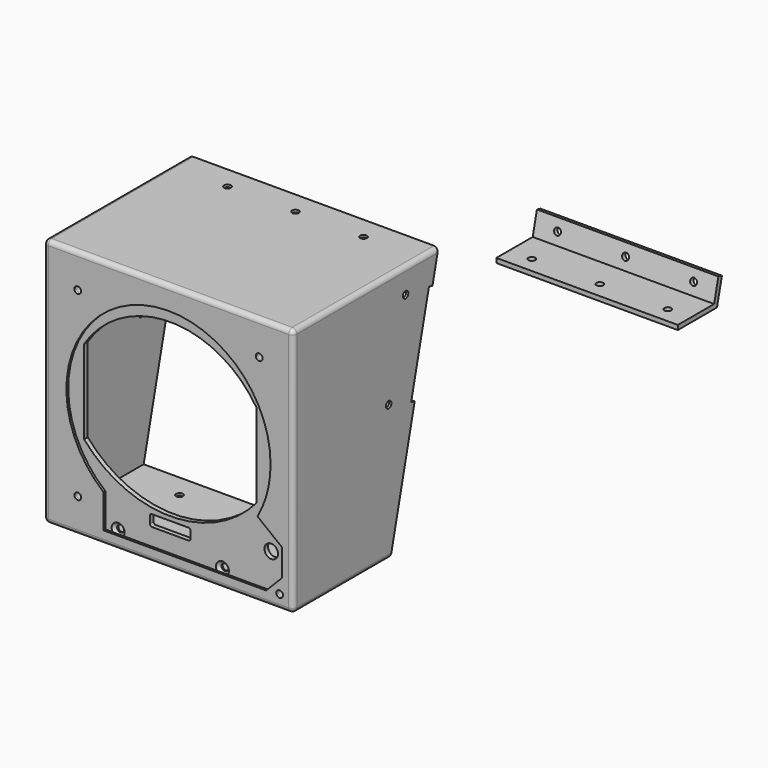
from build123d import *

# Parameters (mm, degrees)
F0_W            = 110
F0_H            = 110
F1_DEPTH        = 60
F2_T            = -1
F3_R            = 1.5
F4_DEPTH        = 110
F5_R            = 2
F6_R            = 1.5
F7_DEPTH        = 1
F8_W            = 106
F8_H            = 106
F8_R            = 1.5
F8_R_2          = 3
F9_DEPTH        = 2
F12_D           = 3
F12_CSINK_D     = 5.7
F12_CSINK_ANGLE = 90
F13_R           = 1.5
F14_R           = 1.5
F15_DEPTH       = 2
F16_DEPTH       = 2
F18_DEPTH       = 40
F21_D           = 3
F21_ON_F19_D    = 3


with BuildPart() as f1:
    # F0 (on Front) → F1 (new body, symmetric)
    with BuildSketch(Plane.XZ):
        with Locations((-111.8381246924, 0)):
            Rectangle(F0_W, F0_H)
    extrude(amount=F1_DEPTH, both=True)

    # F2
    f2_openings = [f1.faces().sort_by_distance(p)[0] for p in [
        (-111.838125, 60, 0),
    ]]
    offset(amount=F2_T, openings=f2_openings)

    # F3 (on face) → F4 (cut)
    with BuildSketch(Plane(origin=(-166.8381246924, 0, 0), x_dir=(0, -1, 0), z_dir=(-1, 0, 0))):
        Polygon((-16.731764906, 41.3868211144), (-20, 55), (-89.8332582524, 55), (-89.8332582524, -55), (6.4086634988, -55), (-6.9270596241, 0.5472844577), align=None)
        Polygon((-14.7870250652, 41.8537118421), (-16.731764906, 41.3868211144), (-6.9270596241, 0.5472844577), (-4.9823197833, 1.0141751854), align=None)
        with Locations((-1.9127707362, 43.9161316519)):
            Circle(F3_R)
        with Locations((7.425043818, 5.021334836)):
            Circle(F3_R)
    extrude(amount=-F4_DEPTH, mode=Mode.SUBTRACT)

    # F5
    f5_edges = [f1.edges().sort_by_distance(p)[0] for p in [
        (-166.838125, -60, 0),
        (-166.838125, -20, 55),
        (-111.838125, -60, 55),
        (-56.838125, -60, 0),
        (-56.838125, -20, 55),
        (-111.838125, -60, -55),
        (-56.838125, -33.204332, -55),
        (-166.838125, -33.204332, -55),
    ]]
    fillet(f5_edges, radius=F5_R)

    # F6 (on face) → F7 (cut)
    with BuildSketch(Plane.XZ.offset(60)):
        with BuildLine():
            ThreePointArc((-72.5995414842, -22.0302879648), (-68.3022989602, -11.3855995808), (-66.8381246924, 0))
            ThreePointArc((-66.8381246924, 0), (-131.0705335784, 40.6830978226), (-140.3987668455, -34.7748432032))
            ThreePointArc((-140.3987668455, -34.7748432032), (-103.5248504668, -44.2254391911), (-72.5995414842, -22.0302879648))
        make_face()
        with BuildLine():
            ThreePointArc((-72.5995414842, -22.0302879648), (-103.5248504668, -44.2254391911), (-140.3987668455, -34.7748432032))
            Line((-140.3987668455, -34.7748432032), (-140.3987668455, -49.5418331784))
            Line((-140.3987668455, -49.5418331784), (-68.7907829881, -49.5418331784))
            Line((-68.7907829881, -49.5418331784), (-61.8381246924, -42.4792694113))
            Line((-61.8381246924, -42.4792694113), (-61.8381246924, -30.4792694113))
            Line((-61.8381246924, -30.4792694113), (-72.5995414842, -22.0302879648))
        make_face()
        with Locations((-151.8381246924, 40)):
            Circle(F6_R)
        with Locations((-71.8381246924, 40)):
            Circle(F6_R)
        with Locations((-151.8381246924, -40)):
            Circle(F6_R)
        with Locations((-62.8381246924, -49)):
            Circle(F6_R)
    extrude(amount=-F7_DEPTH, mode=Mode.SUBTRACT)

    # F13 (on face) + F14 (on face) → F15 (cut)
    with BuildSketch(Plane.XY.offset(55)):
        with Locations((-141.8381246924, 10)):
            Circle(F13_R)
        with Locations((-81.8381246924, 10)):
            Circle(F13_R)
        with Locations((-111.8381246924, 10)):
            Circle(F13_R)
    with BuildSketch(Plane(origin=(0, 0, -55), x_dir=(1, 0, 0), z_dir=(0, 0, -1))):
        with Locations((-141.8381246924, 16.4086634988)):
            Circle(F14_R)
        with Locations((-81.8381246924, 16.4086634988)):
            Circle(F14_R)
        with Locations((-111.8381246924, 16.4086634988)):
            Circle(F14_R)
    extrude(amount=-F15_DEPTH, dir=(0, 0, 1), mode=Mode.SUBTRACT)

    # F14 (on face) → F16 (cut)
    with BuildSketch(Plane(origin=(0, 0, -55), x_dir=(1, 0, 0), z_dir=(0, 0, -1))):
        with Locations((-141.8381246924, 16.4086634988)):
            Circle(F14_R)
        with Locations((-81.8381246924, 16.4086634988)):
            Circle(F14_R)
        with Locations((-111.8381246924, 16.4086634988)):
            Circle(F14_R)
    extrude(amount=-F16_DEPTH, mode=Mode.SUBTRACT)


with BuildPart() as f9:
    # F8 (on face) → F9 (new body)
    with BuildSketch(Plane(origin=(0, -59, 0), x_dir=(-1, 0, 0), z_dir=(0, 1, 0))):
        with Locations((111.8381246924, 0)):
            Rectangle(F8_W, F8_H)
        with Locations((62.8381246924, -49)):
            Circle(F8_R, mode=Mode.SUBTRACT)
        with Locations((67.3356056213, -34.2727303505)):
            Circle(F8_R_2, mode=Mode.SUBTRACT)
        with BuildLine():
            ThreePointArc((102.8381246924, -37.9462198019), (103.1310179113, -37.2391130207), (103.8381246924, -36.9462198019))
            Line((103.8381246924, -36.9462198019), (119.8381246924, -36.9462198019))
            ThreePointArc((119.8381246924, -36.9462198019), (120.5452314736, -37.2391130207), (120.8381246924, -37.9462198019))
            Line((120.8381246924, -37.9462198019), (120.8381246924, -40.9462198019))
            ThreePointArc((120.8381246924, -40.9462198019), (120.5452314736, -41.6533265831), (119.8381246924, -41.9462198019))
            Line((119.8381246924, -41.9462198019), (103.8381246924, -41.9462198019))
            ThreePointArc((103.8381246924, -41.9462198019), (103.1310179113, -41.6533265831), (102.8381246924, -40.9462198019))
            Line((102.8381246924, -40.9462198019), (102.8381246924, -37.9462198019))
        make_face(mode=Mode.SUBTRACT)
        with Locations((151.8381246924, -40)):
            Circle(F8_R, mode=Mode.SUBTRACT)
        with Locations((71.8381246924, 40)):
            Circle(F8_R, mode=Mode.SUBTRACT)
        with BuildLine():
            Line((73.8381246924, -17.6337056415), (73.8381246924, 19.3662943585))
            ThreePointArc((73.8381246924, 19.3662943585), (111.8381246924, 40.2623527721), (149.8381246924, 19.3662943585))
            Line((149.8381246924, 19.3662943585), (149.8381246924, -17.6337056415))
            ThreePointArc((149.8381246924, -17.6337056415), (111.8381246924, -35.1375520229), (73.8381246924, -17.6337056415))
        make_face(mode=Mode.SUBTRACT)
        with Locations((151.8381246924, 40)):
            Circle(F8_R, mode=Mode.SUBTRACT)
    extrude(amount=F9_DEPTH)

    # F12 (through all)
    with Locations(Plane.XZ.offset(59)):
        with Locations((-134.8381246924, -48), (-88.8381246924, -48), (-159.8381246924, 48), (-63.8381246924, 48), (-159.8381246924, 0), (-63.8381246924, 0)):
            CounterSinkHole(F12_D / 2, F12_CSINK_D / 2, counter_sink_angle=F12_CSINK_ANGLE)


with BuildPart() as f18:
    # F17 (on Right) → F18 (new body, symmetric)
    with BuildSketch(Plane.YZ):
        Polygon((52.4713784819, 49.9379689601), (55.1738990921, 61.1947774364), (53.2291592513, 61.6616681641), (50.8947056127, 51.9379689601), (30.8947056127, 51.9379689601), (30.8947056127, 49.9379689601), align=None)
    extrude(amount=F18_DEPTH, both=True)

    # F21 (through all)
    with Locations(Plane(origin=(0, 36.3314379383, -8.7224065358), x_dir=(1, 0, 0), z_dir=(0, -0.9723699204, 0.2334453639))):
        with Locations((-30, 67.3840518135), (0, 67.3840518135), (30, 67.3840518135)):
            Hole(F21_D / 2)

    # F21 on F19 (through all)
    with Locations(Plane.XY.offset(51.9379689601)):
        with Locations((-30, 37.8947056127), (0, 37.8947056127), (30, 37.8947056127)):
            Hole(F21_ON_F19_D / 2)


solid = Compound([f1.part, f9.part, f18.part])
